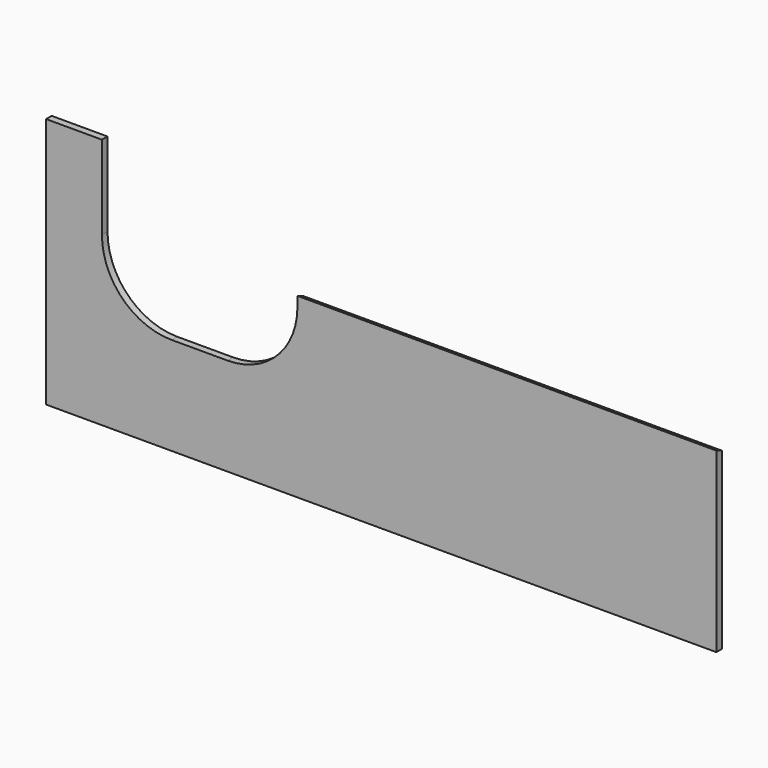
from build123d import *

# Parameters (mm, degrees)
F1_DEPTH = 12.7
F3_DEPTH = 762


# Not quite as in the source:
# - a feature names something its author has since deleted; it is built from what else it names


with BuildPart() as f1:
    # F0 (on Front) → F1 (new body)
    with BuildSketch(Plane.XZ):
        with BuildLine():
            Line((-457.2, 0), (0, 0))
            Line((0, 0), (762, 0))
            Line((762, 0), (762, 317.5))
            Line((762, 317.5), (0, 317.5))
            Line((0, 317.5), (0, 304.8))
            ThreePointArc((0, 304.8), (-37.1974387893, 214.9974387893), (-127, 177.8))
            Line((-127, 177.8), (-228.6, 177.8))
            ThreePointArc((-228.6, 177.8), (-318.4025612107, 214.9974387893), (-355.6, 304.8))
            Line((-355.6, 304.8), (-355.6, 457.2))
            Line((-355.6, 457.2), (-457.2, 457.2))
            Line((-457.2, 457.2), (-457.2, 0))
        make_face()
    extrude(amount=F1_DEPTH)

    # F2 (on face) → F3 (join, through all)
    with BuildSketch(Plane.YZ.offset(762)):
        Polygon((-12.7, 317.5), (0, 317.5), (-12.7, 322.7605122421), align=None)
    extrude(amount=-F3_DEPTH)


solid = f1.part
